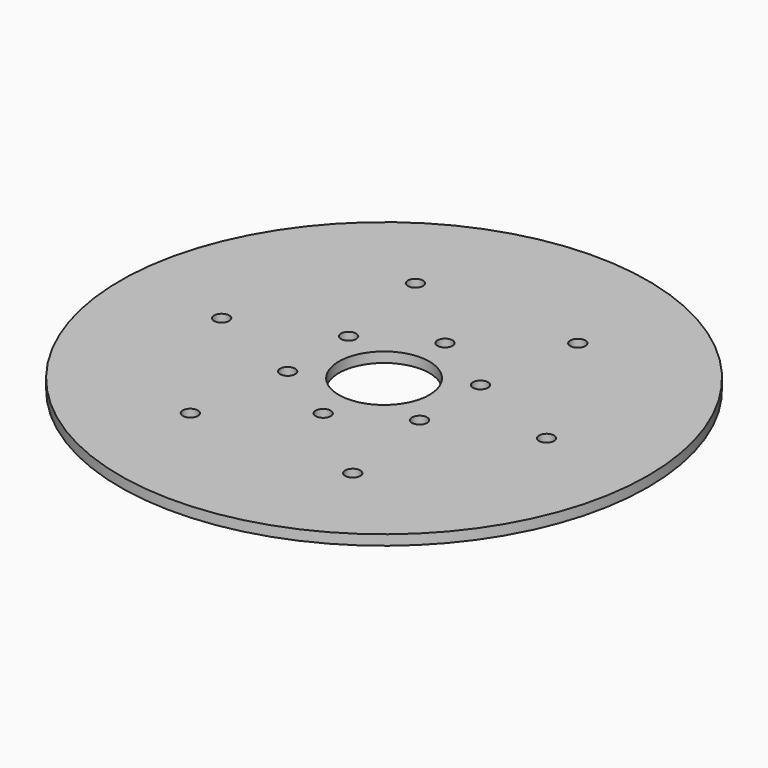
from build123d import *

# Parameters (mm, degrees)
F0_R            = 82.55
F0_R_2          = 14.1605
F1_DEPTH        = 3.175
F2_R            = 2.3622
F3_DEPTH        = 3.176
F3_COPIES_COUNT = 6


# Not quite as in the source:
# - a pattern or mirror of a feature is missing from the dataset's text; its kind, count and spacing are read off the source's solid


with BuildPart() as f1:
    # F0 (on Top) → F1 (new body)
    with BuildSketch(Plane.XY):
        Circle(F0_R)
        Circle(F0_R_2, mode=Mode.SUBTRACT)
    extrude(amount=F1_DEPTH)

    # F2 (on face) → F3 (cut, through all)
    with BuildSketch(Plane.XY.offset(3.175)):
        with Locations((0, 23.8125)):
            Circle(F2_R)
        with Locations((25.4, 43.9940905122)):
            Circle(F2_R)
    f3 = extrude(amount=-F3_DEPTH, mode=Mode.SUBTRACT)

    # F3_copies: F3 ×6 about axis
    f3_copies_axis = Axis((0, 0, 0), (0, 0, 1))
    for i in range(1, F3_COPIES_COUNT):
        add(f3.rotate(f3_copies_axis, i * 360 / F3_COPIES_COUNT), mode=Mode.SUBTRACT)


solid = f1.part
